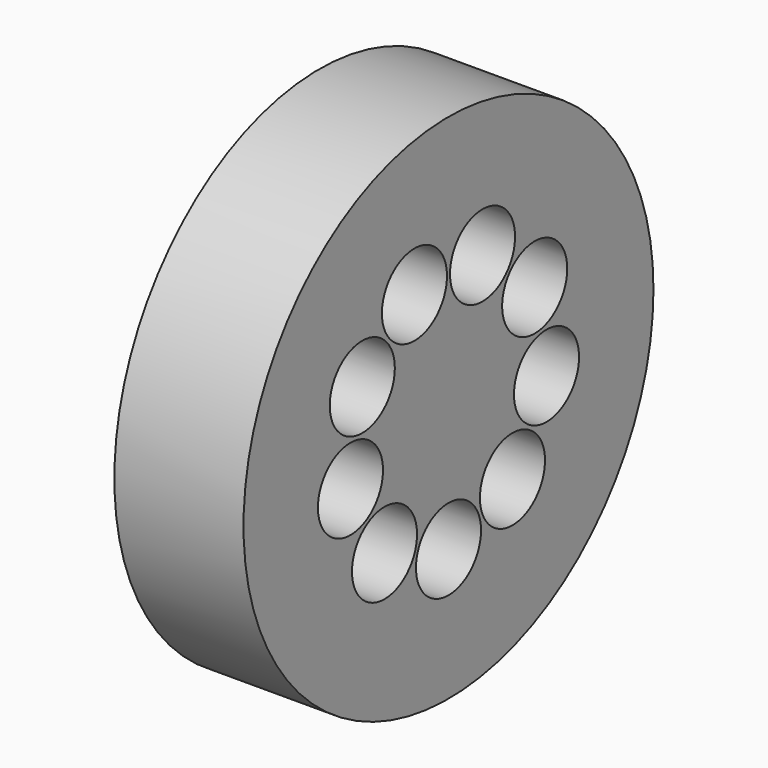
from build123d import *

# Parameters (mm, degrees)
F0_R            = 50.3734102362
F1_DEPTH        = 25.4
F2_R            = 7.9966512346
F3_DEPTH        = 25.4
F3_COPIES_COUNT = 9


# Not quite as in the source:
# - a pattern or mirror of a feature is missing from the dataset's text; its kind, count and spacing are read off the source's solid


with BuildPart() as f1:
    # F0 (on Right) → F1 (new body)
    with BuildSketch(Plane.YZ):
        Circle(F0_R)
    extrude(amount=F1_DEPTH)

    # F2 (on face) → F3 (cut)
    with BuildSketch(Plane.YZ.offset(25.4)):
        with Locations((0, -24.4634896517)):
            Circle(F2_R)
    f3 = extrude(amount=-F3_DEPTH, mode=Mode.SUBTRACT)

    # F3_copies: F3 ×9 about axis
    f3_copies_axis = Axis((0, 0, 0), (1, 0, 0))
    for i in range(1, F3_COPIES_COUNT):
        add(f3.rotate(f3_copies_axis, i * 360 / F3_COPIES_COUNT), mode=Mode.SUBTRACT)


solid = f1.part
